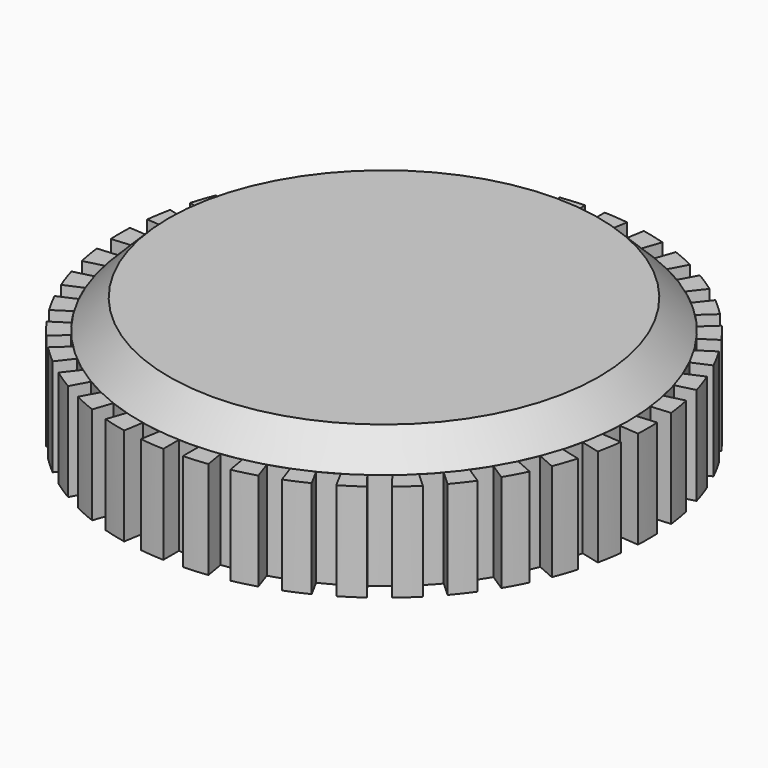
from build123d import *

# Parameters (mm, degrees)
F0_R            = 13.5
F1_DEPTH        = 5
F2_R            = 12.5
F3_DEPTH        = 1.5
F5_DEPTH        = 25
F5_COPIES_COUNT = 38
F6_SIZE         = 1.49999
F7_R            = 1.55
F8_DEPTH        = 3


# Not quite as in the source:
# - a fillet or chamfer is up to 0.001 mm smaller than in the source, because OpenCascade refuses the exact size
# - a pattern or mirror of a feature is missing from the dataset's text; its kind, count and spacing are read off the source's solid


with BuildPart() as f1:
    # F0 (on Top) → F1 (new body)
    with BuildSketch(Plane.XY):
        Circle(F0_R)
    extrude(amount=F1_DEPTH)

    # F2 (on face) → F3 (join)
    with BuildSketch(Plane.XY.offset(5)):
        Circle(F2_R)
    extrude(amount=F3_DEPTH)

    # F4 (on face) → F5 (cut)
    with BuildSketch(Plane.XY.offset(5)):
        with BuildLine():
            ThreePointArc((0.5, 13.4907375632), (0, 13.5), (-0.5, 13.4907375632))
            Line((-0.5, 13.4907375632), (-0.5, 12.4899959968))
            ThreePointArc((-0.5, 12.4899959968), (0, 12.5), (0.5, 12.4899959968))
            Line((0.5, 12.4899959968), (0.5, 13.4907375632))
        make_face()
    f5 = extrude(amount=-F5_DEPTH, mode=Mode.SUBTRACT)

    # F5_copies: F5 ×38 about axis
    f5_copies_axis = Axis((0, 0, 0), (0, 0, 1))
    for i in range(1, F5_COPIES_COUNT):
        add(f5.rotate(f5_copies_axis, i * 360 / F5_COPIES_COUNT), mode=Mode.SUBTRACT)

    # F6 (size 1.5 in the source; OpenCascade refuses exactly that, so slightly less here)
    f6_edges = [f1.edges().sort_by_distance(p)[0] for p in [
        (-12.5, 0, 6.5),
    ]]
    chamfer(f6_edges, length=F6_SIZE)

    # F7 (on face) → F8 (cut)
    with BuildSketch(Plane(origin=(0, 0, 0), x_dir=(1, 0, 0), z_dir=(0, 0, -1))):
        Circle(F7_R)
    extrude(amount=-F8_DEPTH, mode=Mode.SUBTRACT)


solid = f1.part
